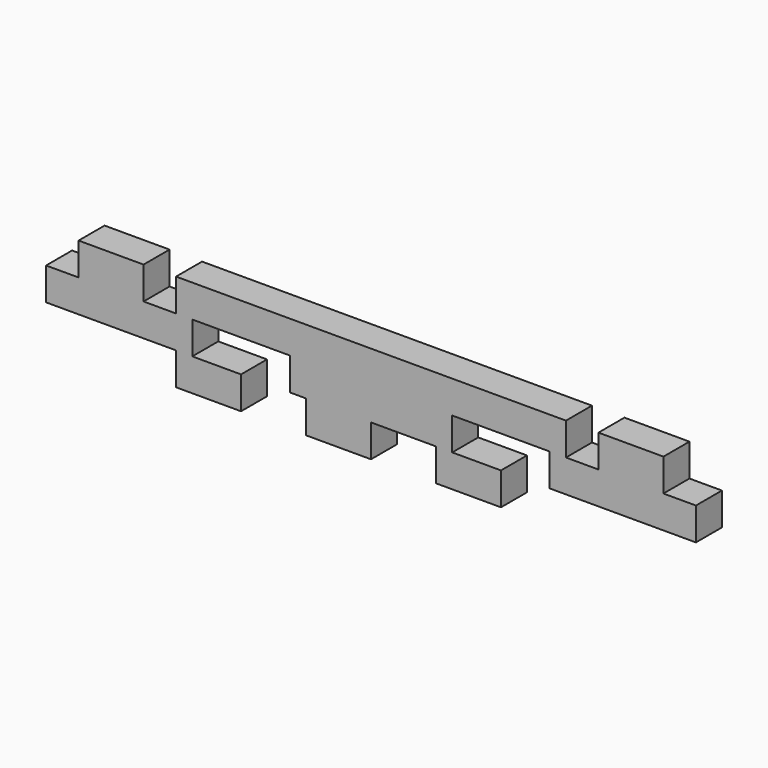
from build123d import *

# Parameters (mm, degrees)
F0_W     = 6.35
F0_H     = 6.35
F0_W_2   = 12.7
F1_DEPTH = 6.35


# Not quite as in the source:
# - a feature names something its author has since deleted; it is built from what else it names


with BuildPart() as f1:
    # F0 (on Front) → F1 (new body)
    with BuildSketch(Plane.XZ):
        Polygon((38.1, 3.175), (38.1, 9.525), (-38.1, 9.525), (-38.1, 3.175), (-38.1, -3.175), (-34.925, -3.175), (-34.925, 3.175), (-15.875, 3.175), (-15.875, -3.175), (-12.7, -3.175), (0, -3.175), (12.7, -3.175), (15.875, -3.175), (15.875, 3.175), (34.925, 3.175), (34.925, -3.175), (38.1, -3.175), align=None)
        Polygon((-44.45, 3.175), (-44.45, 9.525), (-57.15, 9.525), (-57.15, 3.175), (-57.15, -3.175), (-44.45, -3.175), align=None)
        with Locations((-60.325, 0)):
            Rectangle(F0_W, F0_H)
        with Locations((-41.275, 0)):
            Rectangle(F0_W, F0_H)
        with Locations((41.275, 0)):
            Rectangle(F0_W, F0_H)
        with Locations((60.325, 0)):
            Rectangle(F0_W, F0_H)
        Polygon((57.15, 3.175), (57.15, 9.525), (44.45, 9.525), (44.45, 3.175), (44.45, -3.175), (57.15, -3.175), align=None)
        Polygon((-34.925, -3.175), (-38.1, -3.175), (-38.1, -9.525), (-25.4, -9.525), (-25.4, -3.175), align=None)
        with Locations((-6.35, -6.35)):
            Rectangle(F0_W_2, F0_H)
        Polygon((12.7, -9.525), (25.4, -9.525), (25.4, -3.175), (19.05, -3.175), (15.875, -3.175), (12.7, -3.175), align=None)
    extrude(amount=F1_DEPTH)


solid = f1.part
